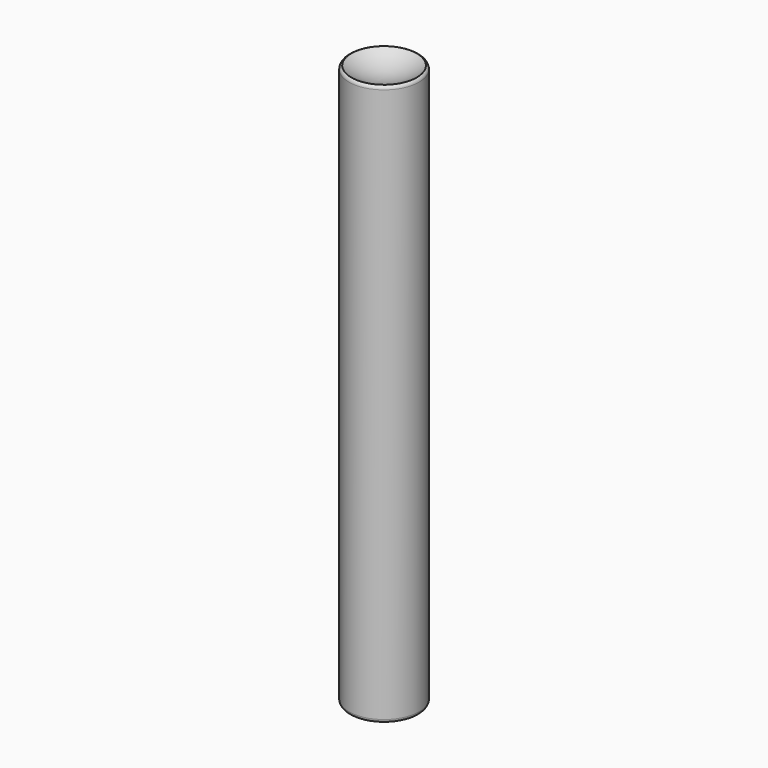
from build123d import *

# Parameters (mm, degrees)
F0_R          = 5
F1_DEPTH      = 40
F1_DEPTH_BACK = 40


# Not quite as in the source:
# - a fillet or chamfer that OpenCascade refuses, or shapes differently, is made with other operations: its cross-section is extruded or revolved along the edge and cut away or added
# - a pattern or mirror of a feature is missing from the dataset's text; its kind, count and spacing are read off the source's solid


with BuildPart() as f1:
    # F0 (on Top) → F1 (new body, two sides)
    with BuildSketch(Plane.XY) as f1_sk:
        Circle(F0_R)
    extrude(amount=F1_DEPTH)
    extrude(f1_sk.sketch, amount=-F1_DEPTH_BACK)

    # F2 (on Right) → F3 (revolve, cut)
    with BuildSketch(Plane.YZ):
        with BuildLine():
            Line((0, 38.5), (0, 54.5))
            ThreePointArc((0, 54.5), (-8, 46.5), (0, 38.5))
        make_face()
    f3 = revolve(axis=Axis((0, 0, 46.5), (0, 0, -1)), mode=Mode.SUBTRACT)

    # F3_copies: F3 across plane
    add(f3.mirror(Plane(origin=(0, 0, 0), x_dir=(-1, 0, 0), z_dir=(0, 0, -1))), mode=Mode.SUBTRACT)

    # F4: fillet of radius 0.5 on 2 edges, made by hand

    # F4_s1 → F4_t2 (revolve, cut)
    with BuildSketch(Plane.XZ):
        with BuildLine():
            ThreePointArc((5, -39.5275534539), (4.9073357112, -39.8175148623), (4.6636895265, -40))
            Line((4.6636895265, -40), (4.6669633171, -40.0094489309))
            ThreePointArc((4.6669633171, -40.0094489309), (4.8318447633, -40.01), (5, -40.01))
            Line((5, -40.01), (5.01, -40))
            Line((5.01, -40), (5.01, -39.5275534539))
            Line((5.01, -39.5275534539), (5, -39.5275534539))
        make_face()
    revolve(axis=Axis((0, 0, -40), (0, 0, 1)), mode=Mode.SUBTRACT)

    # F4_s3 → F4_t4 (revolve, cut)
    with BuildSketch(Plane.XZ):
        with BuildLine():
            ThreePointArc((5, 39.5275534539), (4.9073357112, 39.8175148623), (4.6636895265, 40))
            Line((4.6636895265, 40), (4.6669633171, 40.0094489309))
            ThreePointArc((4.6669633171, 40.0094489309), (4.8318447633, 40.01), (5, 40.01))
            Line((5, 40.01), (5.01, 40))
            Line((5.01, 40), (5.01, 39.5275534539))
            Line((5.01, 39.5275534539), (5, 39.5275534539))
        make_face()
    revolve(axis=Axis((0, 0, 40), (0, 0, 1)), mode=Mode.SUBTRACT)


solid = f1.part
